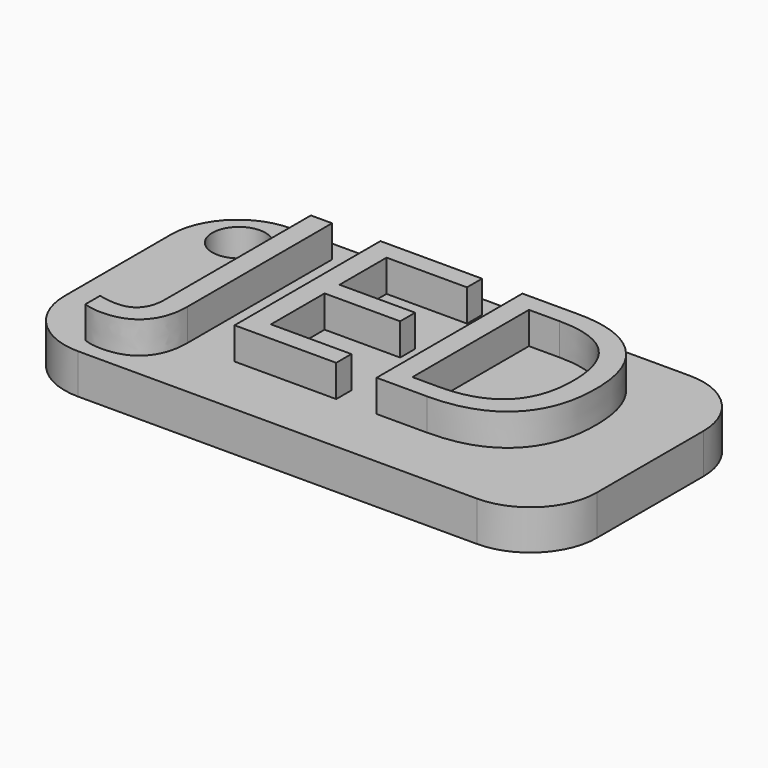
from build123d import *

# Parameters (mm, degrees)
F0_W         = 40
F0_H         = 20
F1_DEPTH     = 3
F2_TEXT_SIZE = 19.1895776273
F3_DEPTH     = 2.4
F4_R         = 5
F6_D         = 4


# Not quite as in the source:
# - Text() gives the source's letters only with a copy of the font that has no kerning and outlines rounded to 1/6400 em; it was checked with that copy


with BuildPart() as f1:
    # F0 (on Top) → F1 (new body)
    with BuildSketch(Plane.XY):
        with Locations((20, 10)):
            Rectangle(F0_W, F0_H)
    extrude(amount=F1_DEPTH)

    # F2 (on face) → F3 (join)
    with BuildSketch(Plane.XY.offset(3)):
        with Locations((5.991341779, 4.7169891186)):
            Text('JED', F2_TEXT_SIZE, font='Open Sans', text_align=(TextAlign.LEFT, TextAlign.BOTTOM))
    extrude(amount=F3_DEPTH)

    # F4
    f4_edges = [f1.edges().sort_by_distance(p)[0] for p in [
        (40, 0, 1.5),
        (40, 20, 1.5),
        (0, 20, 1.5),
        (0, 0, 1.5),
    ]]
    fillet(f4_edges, radius=F4_R)

    # F6 (through all)
    with Locations(Plane.XY.offset(3)):
        with Locations((3.7573953159, 16.6757758707)):
            Hole(F6_D / 2)


solid = f1.part
